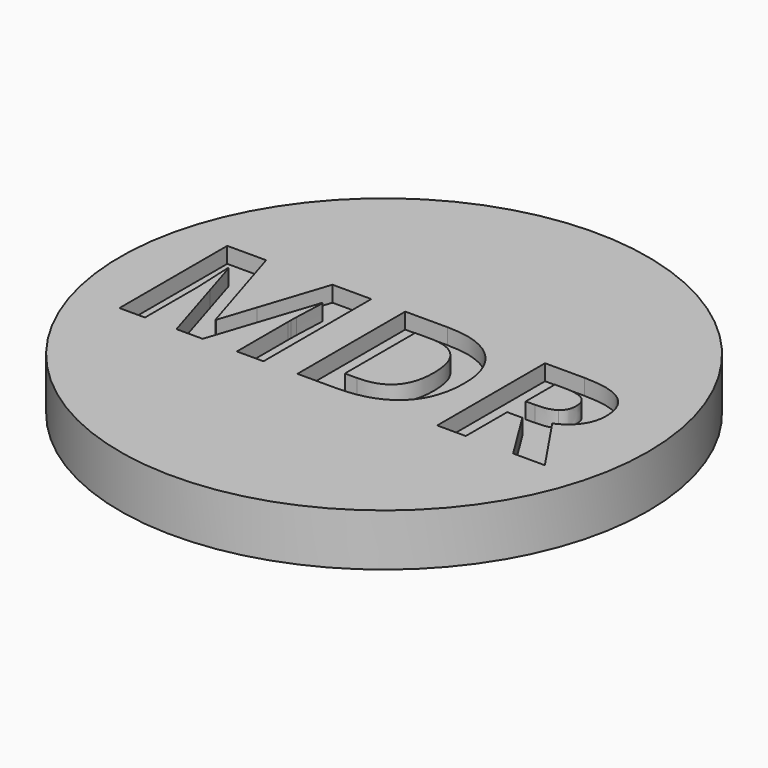
from build123d import *

# Parameters (mm, degrees)
F0_R     = 11.65
F1_DEPTH = 2.3
F3_DEPTH = 0.7


with BuildPart() as f1:
    # F0 (on Top) → F1 (new body)
    with BuildSketch(Plane.XY):
        Circle(F0_R)
    extrude(amount=F1_DEPTH)

    # F2 (on face) → F3 (cut)
    with BuildSketch(Plane.XY.offset(2.3)):
        with BuildLine():
            Line((-9.2821657193, 2.94921875), (-9.2821657193, 0))
            Line((-9.2821657193, 0), (-8.1577947596, 0))
            add(Edge.make_bspline(
                [(-8.2326865526, 1.6666666667), (-8.1704547679, 0.5330109879), (-8.1577947596, 0)],
                knots=[0, 0, 0, 0.7965668448, 0.7965668448, 0.7965668448], degree=2))
            Line((-8.2326865526, 1.6666666667), (-8.1962282193, 1.6666666667))
            Line((-8.1962282193, 1.6666666667), (-7.6846954812, 0))
            Line((-7.6846954812, 0), (-6.6522663233, 0))
            Line((-6.6522663233, 0), (-7.5647178026, 2.94921875))
            Line((-7.5647178026, 2.94921875), (-9.2821657193, 2.94921875))
        make_face()
        with BuildLine():
            Line((-8.1577947596, 0), (-9.2821657193, 0))
            Line((-9.2821657193, 0), (-9.2821657193, -3))
            Line((-9.2821657193, -3), (-8.1545615526, -3))
            Line((-8.1545615526, -3), (-8.1545615526, -0.2330729167))
            add(Edge.make_bspline(
                [(-8.1577947596, 0), (-8.1545615526, -0.1361243036), (-8.1545615526, -0.2330729167)],
                knots=[0.7965668448, 0.7965668448, 0.7965668448, 1, 1, 1], degree=2))
        make_face()
        Polygon((-5.6076865526, -3), (-4.6199839255, 0), (-5.607097373, 0), (-6.132426136, -1.6002604167), (-6.1571657193, -1.6002604167), (-6.6522663233, 0), (-7.6846954812, 0), (-6.7639365526, -3), align=None)
        with BuildLine():
            Line((-4.0973563741, 0), (-2.9227907193, 0))
            Line((-2.9227907193, 0), (-2.9227907193, 2.94921875))
            Line((-2.9227907193, 2.94921875), (-4.6389365526, 2.94921875))
            Line((-4.6389365526, 2.94921875), (-5.607097373, 0))
            Line((-5.607097373, 0), (-4.6199839255, 0))
            Line((-4.6199839255, 0), (-4.073832386, 1.6588541667))
            Line((-4.073832386, 1.6588541667), (-4.0373740526, 1.6588541667))
            add(Edge.make_bspline(
                [(-4.0920615526, 0.2760416667), (-4.085551136, 0.5364583333), (-4.0373740526, 1.6588541667)],
                knots=[0, 0, 0, 1, 1, 1], degree=2))
            add(Edge.make_bspline(
                [(-4.0973563741, 0), (-4.0957587805, 0.1281525523), (-4.0920615526, 0.2760416667)],
                knots=[0.432105801, 0.432105801, 0.432105801, 1, 1, 1], degree=2))
        make_face()
        with BuildLine():
            Line((-2.9227907193, -3), (-2.9227907193, 0))
            Line((-2.9227907193, 0), (-4.0973563741, 0))
            add(Edge.make_bspline(
                [(-4.0985719693, -0.18359375), (-4.0985719693, -0.0975101725), (-4.0973563741, 0)],
                knots=[0, 0, 0, 0.432105801, 0.432105801, 0.432105801], degree=2))
            Line((-4.0985719693, -0.18359375), (-4.0985719693, -3))
            Line((-4.0985719693, -3), (-2.9227907193, -3))
        make_face()
        Polygon((-1.425394886, 0), (-0.163676136, 0), (-0.163676136, 1.9153645833), (0, 1.9153645833), (0, 2.94921875), (-1.425394886, 2.94921875), align=None)
        with BuildLine():
            Line((-0.163676136, -1.9583333333), (-0.163676136, 0))
            Line((-0.163676136, 0), (-1.425394886, 0))
            Line((-1.425394886, 0), (-1.425394886, -3))
            Line((-1.425394886, -3), (0.2595009474, -3))
            add(Edge.make_bspline(
                [(2.674214489, -2.21875), (1.8376259474, -3), (0.2595009474, -3)],
                knots=[0, 0, 0, 1, 1, 1], degree=2))
            add(Edge.make_bspline(
                [(3.5108030307, 0.03125), (3.5108030307, -1.4375), (2.674214489, -2.21875)],
                knots=[0, 0, 0, 1, 1, 1], degree=2))
            add(Edge.make_bspline(
                [(2.7048134474, 2.1803385417), (3.5108030307, 1.4114583333), (3.5108030307, 0.03125)],
                knots=[0, 0, 0, 1, 1, 1], degree=2))
            add(Edge.make_bspline(
                [(0.441792614, 2.94921875), (1.898823864, 2.94921875), (2.7048134474, 2.1803385417)],
                knots=[0, 0, 0, 1, 1, 1], degree=2))
            Line((0.441792614, 2.94921875), (0, 2.94921875))
            Line((0, 2.94921875), (0, 1.9153645833))
            Line((0, 1.9153645833), (0.5068967807, 1.9153645833))
            add(Edge.make_bspline(
                [(2.199605114, -0.0013020833), (2.199605114, 1.9153645833), (0.5068967807, 1.9153645833)],
                knots=[0, 0, 0, 1, 1, 1], degree=2))
            add(Edge.make_bspline(
                [(0.3766884474, -1.9583333333), (2.199605114, -1.9583333333), (2.199605114, -0.0013020833)],
                knots=[0, 0, 0, 1, 1, 1], degree=2))
            Line((0.3766884474, -1.9583333333), (-0.163676136, -1.9583333333))
        make_face()
        with BuildLine():
            Line((6.0055946974, -3), (6.0055946974, -0.7174479167))
            Line((6.0055946974, -0.7174479167), (6.676167614, -0.7174479167))
            Line((6.676167614, -0.7174479167), (8.0967405307, -3))
            Line((8.0967405307, -3), (9.496480114, -3))
            add(Edge.make_bspline(
                [(7.746480114, -0.4075520833), (9.090230114, -2.4140625), (9.496480114, -3)],
                knots=[0, 0, 0, 1, 1, 1], degree=2))
            add(Edge.make_bspline(
                [(8.564839489, 0.2330729167), (8.2764280307, -0.17578125), (7.746480114, -0.4075520833)],
                knots=[0, 0, 0, 1, 1, 1], degree=2))
            add(Edge.make_bspline(
                [(8.8532509474, 1.1666666667), (8.8532509474, 0.6419270833), (8.564839489, 0.2330729167)],
                knots=[0, 0, 0, 1, 1, 1], degree=2))
            add(Edge.make_bspline(
                [(8.271870739, 2.5078125), (8.8532509474, 2.06640625), (8.8532509474, 1.1666666667)],
                knots=[0, 0, 0, 1, 1, 1], degree=2))
            add(Edge.make_bspline(
                [(6.476948864, 2.94921875), (7.6904905307, 2.94921875), (8.271870739, 2.5078125)],
                knots=[0, 0, 0, 1, 1, 1], degree=2))
            Line((6.476948864, 2.94921875), (4.7438759474, 2.94921875))
            Line((4.7438759474, 2.94921875), (4.7438759474, -3))
            Line((4.7438759474, -3), (6.0055946974, -3))
        make_face()
        with BuildLine():
            Line((6.4118446974, 0.30859375), (6.0055946974, 0.30859375))
            Line((6.0055946974, 0.30859375), (6.0055946974, 1.9153645833))
            Line((6.0055946974, 1.9153645833), (6.3884071974, 1.9153645833))
            add(Edge.make_bspline(
                [(7.2887978224, 1.736328125), (6.9977821974, 1.9153645833), (6.3884071974, 1.9153645833)],
                knots=[0, 0, 0, 1, 1, 1], degree=2))
            add(Edge.make_bspline(
                [(7.5798134474, 1.1341145833), (7.5798134474, 1.5572916667), (7.2887978224, 1.736328125)],
                knots=[0, 0, 0, 1, 1, 1], degree=2))
            add(Edge.make_bspline(
                [(7.295308239, 0.5078125), (7.5798134474, 0.70703125), (7.5798134474, 1.1341145833)],
                knots=[0, 0, 0, 1, 1, 1], degree=2))
            add(Edge.make_bspline(
                [(6.4118446974, 0.30859375), (7.0108030307, 0.30859375), (7.295308239, 0.5078125)],
                knots=[0, 0, 0, 1, 1, 1], degree=2))
        make_face(mode=Mode.SUBTRACT)
    extrude(amount=-F3_DEPTH, mode=Mode.SUBTRACT)


solid = f1.part
